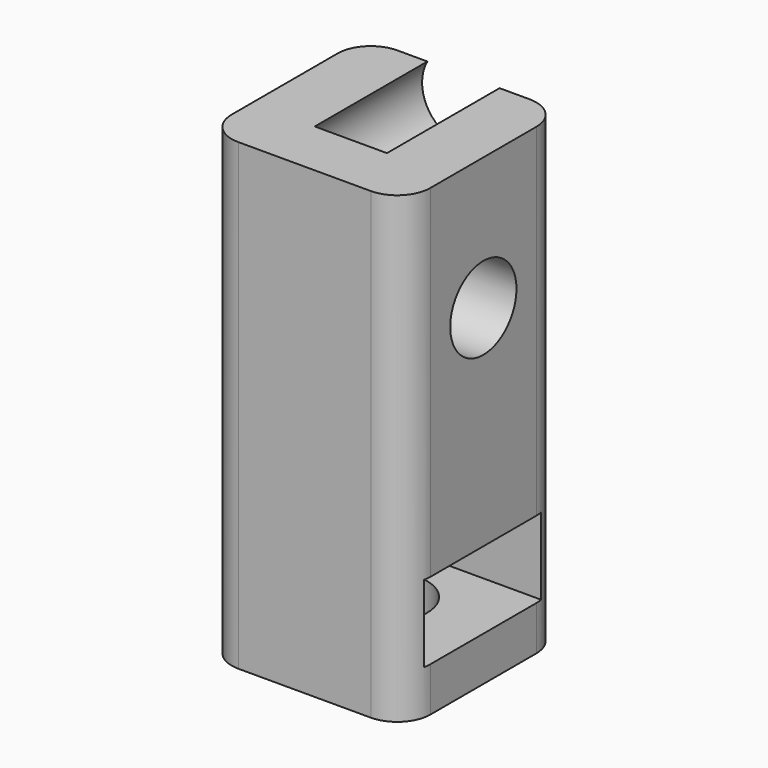
from build123d import *

# Parameters (mm, degrees)
F0_W          = 15.24
F0_H          = 15.24
F1_DEPTH      = 35.56
F2_R          = 3.175
F3_DEPTH      = 12.7
F3_DEPTH_BACK = 3.175
F4_R          = 3.175
F4_W          = 11.2
F4_H          = 5.9
F5_DEPTH      = 12.7
F6_T1_DEPTH   = 48.26
F7_R          = 3.302
F8_DEPTH      = 6.35


# Not quite as in the source:
# - a fillet or chamfer that OpenCascade refuses, or shapes differently, is made with other operations: its cross-section is extruded or revolved along the edge and cut away or added


with BuildPart() as f1:
    # F0 (on Top) → F1 (new body)
    with BuildSketch(Plane.XY):
        Rectangle(F0_W, F0_H)
    extrude(amount=F1_DEPTH)

    # F2 (on Front) → F3 (cut, two sides)
    with BuildSketch(Plane.XZ) as f3_sk:
        with Locations((0, 34.00425)):
            Circle(F2_R)
    extrude(amount=-F3_DEPTH, mode=Mode.SUBTRACT)
    extrude(f3_sk.sketch, amount=F3_DEPTH_BACK, mode=Mode.SUBTRACT)

    # F4 (on Right) → F5 (cut, symmetric)
    with BuildSketch(Plane.YZ):
        with Locations((0, 25.4)):
            Circle(F4_R)
        with Locations((0, 6.35)):
            Rectangle(F4_W, F4_H)
    extrude(amount=F5_DEPTH, both=True, mode=Mode.SUBTRACT)

    # F6: fillet of radius 2.54 on 4 edges, made by hand

    # F6_s2 → F6_t1 (cut)
    with BuildSketch(Plane.XY.offset(-6.35)):
        with BuildLine():
            ThreePointArc((7.62, 5.08), (6.8760512242, 6.8760512242), (5.08, 7.62))
            Line((5.08, 7.62), (7.62, 7.62))
            Line((7.62, 7.62), (7.62, 5.08))
        make_face()
        with BuildLine():
            ThreePointArc((5.08, -7.62), (6.8760512242, -6.8760512242), (7.62, -5.08))
            Line((7.62, -5.08), (7.62, -7.62))
            Line((7.62, -7.62), (5.08, -7.62))
        make_face()
        with BuildLine():
            ThreePointArc((-7.62, 5.08), (-6.8760512242, 6.8760512242), (-5.08, 7.62))
            Line((-5.08, 7.62), (-7.62, 7.62))
            Line((-7.62, 7.62), (-7.62, 5.08))
        make_face()
        with BuildLine():
            ThreePointArc((-5.08, -7.62), (-6.8760512242, -6.8760512242), (-7.62, -5.08))
            Line((-7.62, -5.08), (-7.62, -7.62))
            Line((-7.62, -7.62), (-5.08, -7.62))
        make_face()
    extrude(amount=F6_T1_DEPTH, mode=Mode.SUBTRACT)

    # F7 (on face) → F8 (cut)
    with BuildSketch(Plane(origin=(0, 0, 0), x_dir=(1, 0, 0), z_dir=(0, 0, -1))):
        Circle(F7_R)
    extrude(amount=-F8_DEPTH, mode=Mode.SUBTRACT)


solid = f1.part
